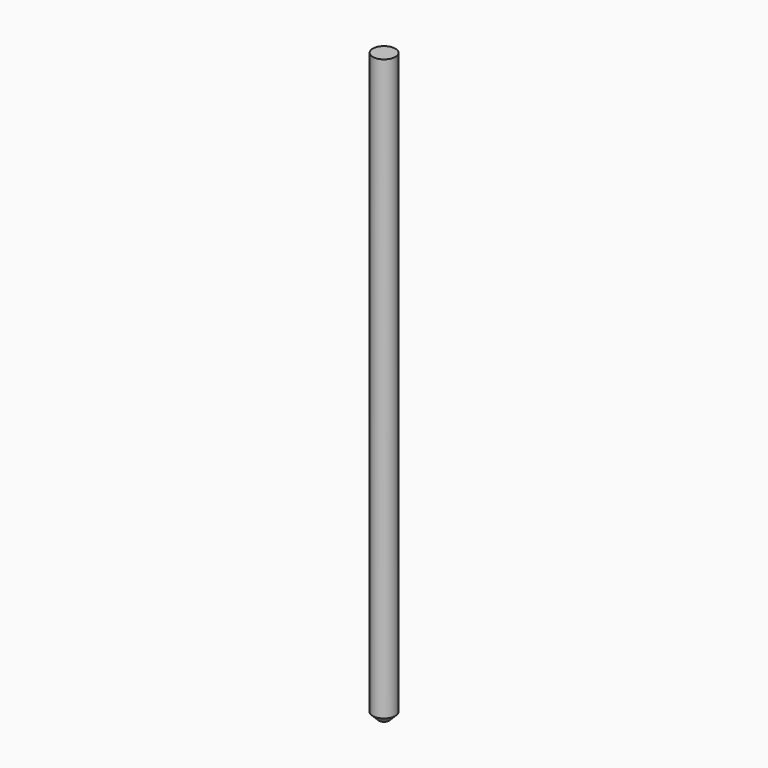
from build123d import *

# Parameters (mm, degrees)
F0_R     = 1.5875
F1_DEPTH = 82.55
F2_SIZE  = 0.889


# Not quite as in the source:
# - a length typed as a fraction of an inch, garbled in the dataset ("3 / 203.2 mm" for 3/8 in), is restored


with BuildPart() as f1:
    # F0 (on Top) → F1 (new body)
    with BuildSketch(Plane.XY):
        Circle(F0_R)
    extrude(amount=-F1_DEPTH)

    # F2
    f2_edges = [f1.edges().sort_by_distance(p)[0] for p in [
        (-1.5875, 0, -82.55),
    ]]
    chamfer(f2_edges, length=F2_SIZE)


solid = f1.part
